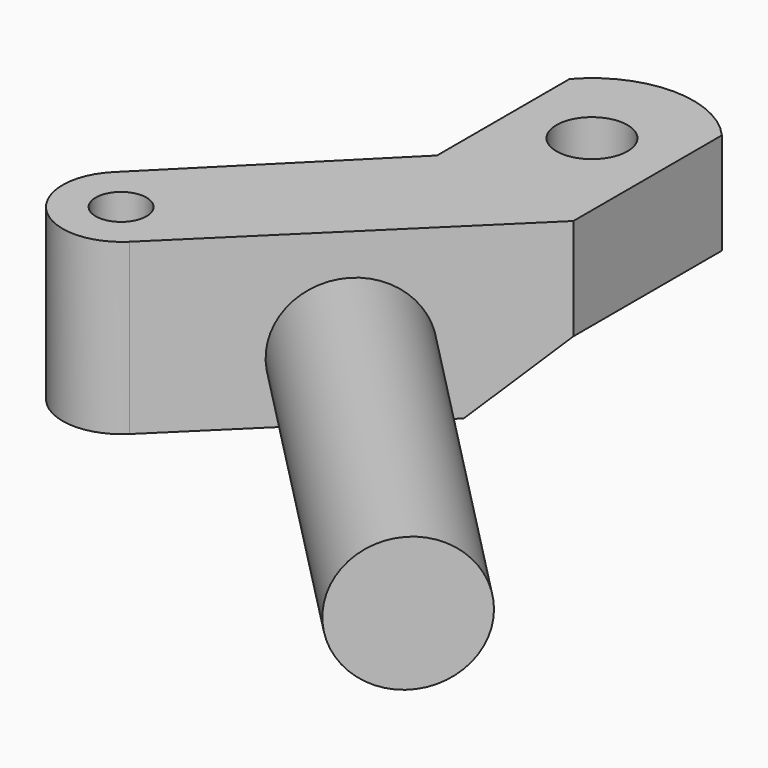
from build123d import *

# Parameters (mm, degrees)
F0_R     = 1.5
F0_R_2   = 2.1
F1_DEPTH = 6
F2_R     = 3.98
F3_DEPTH = 26
F4_R     = 1.5
F5_DEPTH = 4
F6_SIZE  = 3.99999


# Not quite as in the source:
# - a fillet or chamfer is up to 0.001 mm smaller than in the source, because OpenCascade refuses the exact size


with BuildPart() as f1:
    # F0 (on Top) → F1 (new body)
    with BuildSketch(Plane.XY):
        with BuildLine():
            Line((4.5, 0), (4.5, 3.9686269666))
            ThreePointArc((4.5, 3.9686269666), (0, 6), (-4.5, 3.9686269666))
            Line((-4.5, 3.9686269666), (-4.5, 0))
            Line((-4.5, 0), (-4.5, -5.813701588))
            Line((-4.5, -5.813701588), (-15.143203234, -16.4569048219))
            ThreePointArc((-15.143203234, -16.4569048219), (-15.1189316865, -21.3823807428), (-10.1934557657, -21.4066522902))
            Line((-10.1934557657, -21.4066522902), (4.5, -7))
            Line((4.5, -7), (4.5, 0))
        make_face()
        with Locations((-12.6691633098, -18.9323580438)):
            Circle(F0_R, mode=Mode.SUBTRACT)
        Circle(F0_R_2, mode=Mode.SUBTRACT)
    extrude(amount=F1_DEPTH)

    # F2 (on face) → F3 (join)
    with BuildSketch(Plane(origin=(5.7049735344, -5.8185465008, 0), x_dir=(0.7140411723, 0.7001037097, 0), z_dir=(0.7001037097, -0.7140411723, 0))):
        with Locations((-11.9764822387, -0.39)):
            Circle(F2_R)
    extrude(amount=F3_DEPTH)

    # F4 (on face) → F5 (join)
    with BuildSketch(Plane(origin=(0, 0, 0), x_dir=(1, 0, 0), z_dir=(0, 0, -1))):
        with BuildLine():
            ThreePointArc((-10.1934557657, 21.4066522902), (-15.1189316865, 21.3823807428), (-15.143203234, 16.4569048219))
            Line((-15.143203234, 16.4569048219), (-4.5, 5.813701588))
            Line((-4.5, 5.813701588), (4.5, 7))
            Line((4.5, 7), (-10.1934557657, 21.4066522902))
        make_face()
        with Locations((-12.6691633098, 18.9323580438)):
            Circle(F4_R, mode=Mode.SUBTRACT)
    extrude(amount=F5_DEPTH)

    # F6 (size 4 in the source; OpenCascade refuses exactly that, so slightly less here)
    f6_edges = [f1.edges().sort_by_distance(p)[0] for p in [
        (0, -6.406851, -4),
    ]]
    chamfer(f6_edges, length=F6_SIZE)


solid = f1.part
